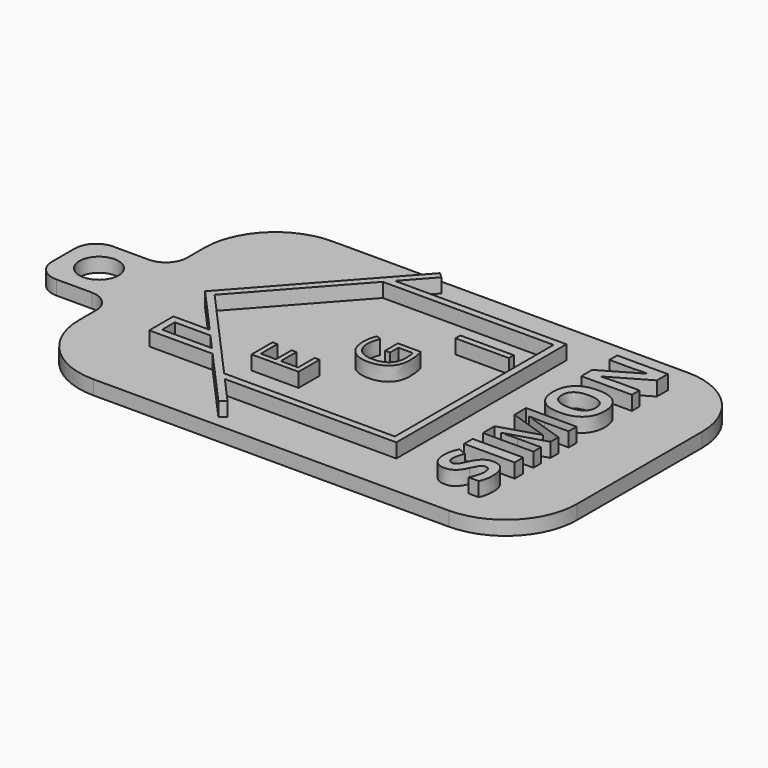
from build123d import *

# Parameters (mm, degrees)
F0_R          = 2.75
F1_DEPTH      = 2
F3_DEPTH      = 2
F4_TEXT_SIZE  = 9.2623043909
F5_DEPTH      = 2
F6_TEXT_SIZE  = 9.2203093628
F7_DEPTH      = 2
F8_TEXT_SIZE  = 10.5208345404
F9_DEPTH      = 2
F10_TEXT_SIZE = 9.9545964454
F11_DEPTH     = 2


# Not quite as in the source:
# - Text() gives the source's letters only with a copy of the font that has no kerning and outlines rounded to 1/6400 em; it was checked with that copy


with BuildPart() as f1:
    # F0 (on Top) → F1 (new body)
    with BuildSketch(Plane.XY):
        with BuildLine():
            ThreePointArc((40, 11), (37.0710678119, 18.0710678119), (30, 21))
            Line((30, 21), (-20, 21))
            ThreePointArc((-20, 21), (-27.0710678119, 18.0710678119), (-30, 11))
            Line((-30, 11), (-30, 8))
            ThreePointArc((-30, 8), (-30.8786796564, 5.8786796564), (-33, 5))
            Line((-33, 5), (-38, 5))
            ThreePointArc((-38, 5), (-40.1213203436, 4.1213203436), (-41, 2))
            Line((-41, 2), (-41, -2))
            ThreePointArc((-41, -2), (-40.1213203436, -4.1213203436), (-38, -5))
            Line((-38, -5), (-33, -5))
            ThreePointArc((-33, -5), (-30.8786796564, -5.8786796564), (-30, -8))
            Line((-30, -8), (-30, -11))
            ThreePointArc((-30, -11), (-27.0710678119, -18.0710678119), (-20, -21))
            Line((-20, -21), (30, -21))
            ThreePointArc((30, -21), (37.0710678119, -18.0710678119), (40, -11))
            Line((40, -11), (40, 11))
        make_face()
        with Locations((-36, 0)):
            Circle(F0_R, mode=Mode.SUBTRACT)
    extrude(amount=F1_DEPTH)

    # F2 (on face) → F3 (join)
    with BuildSketch(Plane.XY.offset(2)):
        Polygon((-2.8916704468, -18.8033767045), (-6.3510161364, -14.9424578995), (17.7639125139, -14.9424578995), (17.7639125139, 0), (17.7639125139, 14.9424578995), (-6.3510161364, 14.9424578995), (-2.8916704468, 18.8033767045), (-3.6364476894, 19.4706898685), (-21.0819963969, 0), (-14.9512048705, -6.8424755484), (-20.0612263978, -6.8424755484), (-20.0612263978, -11.0868465379), (-11.148289754, -11.0868465379), (-3.6364476894, -19.4706898685), align=None)
        Polygon((-19.0612263978, -7.8424755484), (-14.0552145987, -7.8424755484), (-12.0442800258, -10.0868465379), (-19.0612263978, -10.0868465379), align=None, mode=Mode.SUBTRACT)
        Polygon((-7.2470064082, -13.9424578995), (-19.7393130511, 0), (-7.2470064082, 13.9424578995), (16.7639125139, 13.9424578995), (16.7639125139, 0), (16.7639125139, -13.9424578995), align=None, mode=Mode.SUBTRACT)
    extrude(amount=F3_DEPTH)

    # F4 (on face) → F5 (join)
    with BuildSketch(Plane.XY.offset(2)):
        with Locations(Location((-1.1006611987, -9.4460770488), (0, 0, 90))):
            Text('E', F4_TEXT_SIZE, font='Open Sans', text_align=(TextAlign.LEFT, TextAlign.BOTTOM))
    extrude(amount=F5_DEPTH)

    # F6 (on face) → F7 (join)
    with BuildSketch(Plane.XY.offset(2)):
        with Locations(Location((6.6386227412, -2.4920478463), (0, 0, 90))):
            Text('G', F6_TEXT_SIZE, font='Open Sans', text_align=(TextAlign.LEFT, TextAlign.BOTTOM))
    extrude(amount=F7_DEPTH)

    # F8 (on face) → F9 (join)
    with BuildSketch(Plane.XY.offset(2)):
        with Locations(Location((14.8795806671, 7.3962597308), (0, 0, 90))):
            Text('I', F8_TEXT_SIZE, font='Open Sans', text_align=(TextAlign.LEFT, TextAlign.BOTTOM))
    extrude(amount=F9_DEPTH)

    # F10 (on face) → F11 (join)
    with BuildSketch(Plane.XY.offset(2)):
        with Locations(Location((30.8947749436, -16.9348778727), (0, 0, 90))):
            Text('SIMON', F10_TEXT_SIZE, font='Open Sans', font_style=FontStyle.BOLD, text_align=(TextAlign.LEFT, TextAlign.BOTTOM))
    extrude(amount=F11_DEPTH)


solid = f1.part
